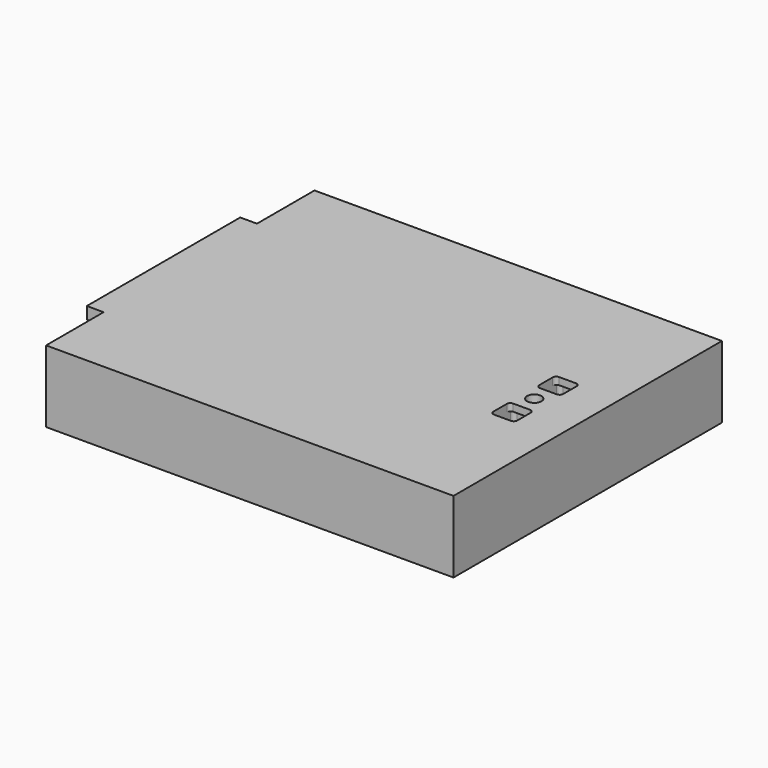
from build123d import *

# Parameters (mm, degrees)
F0_W     = 5
F0_H     = 24
F0_H_2   = 12
F0_R     = 2.55
F0_W_2   = 3
F1_DEPTH = 30
F2_START = -13
F2_DEPTH = 17
F3_START = -3
F3_DEPTH = 27
F4_START = -8
F4_DEPTH = 22
F5_DEPTH = 3
F6_DEPTH = 5


# Not quite as in the source:
# - a feature names something its author has since deleted; it is built from what else it names


with BuildPart() as f1:
    # F0 (on Top) → F1 (new body)
    with BuildSketch(Plane.XY):
        Polygon((82.5, 70), (-87.5, 70), (-87.5, 65), (-87.5, 40), (-87.5, 5), (-87.5, -5), (-87.5, -40), (-87.5, -65), (-87.5, -70), (-82.5, -70), (82.5, -70), (82.5, 0), align=None)
        Polygon((47.5, -65), (-82.5, -65), (-82.5, 65), (47.5, 65), (52.5, 65), (77.5, 65), (77.5, 0), (77.5, -65), (52.5, -65), align=None, mode=Mode.SUBTRACT)
        with BuildLine():
            Line((77.5, 65), (52.5, 65))
            Line((52.5, 65), (52.5, 41))
            Line((52.5, 41), (55.5, 41))
            Line((55.5, 41), (55.5, 44.499418828))
            ThreePointArc((55.5, 44.499418828), (55.9393398282, 45.5600789998), (57, 45.999418828))
            Line((57, 45.999418828), (63.8683293534, 45.999418828))
            ThreePointArc((63.8683293534, 45.999418828), (64.9248818439, 45.5641708343), (65.3682845321, 44.5110146078))
            Line((65.3682845321, 44.5110146078), (65.5, 27.4731523439))
            Line((65.5, 27.4731523439), (65.5, 18.9731523439))
            Line((65.5, 18.9731523439), (65.5, 17.4731523439))
            Line((65.5, 17.4731523439), (65.5, 16.9731523439))
            Line((65.5, 16.9731523439), (65.5, 15.4731523439))
            Line((65.5, 15.4731523439), (65.5, 8.4731523439))
            Line((65.5, 8.4731523439), (65.5, 6.9731523439))
            Line((65.5, 6.9731523439), (65.5, 6.4731523439))
            ThreePointArc((65.5, 6.4731523439), (65.0606601718, 5.4124921721), (64, 4.9731523439))
            Line((64, 4.9731523439), (57, 4.9731523439))
            ThreePointArc((57, 4.9731523439), (55.9393398282, 5.4124921721), (55.5, 6.4731523439))
            Line((55.5, 6.4731523439), (55.5, 6.9731523439))
            Line((55.5, 6.9731523439), (55.5, 8.4731523439))
            Line((55.5, 8.4731523439), (55.5, 15.4731523439))
            Line((55.5, 15.4731523439), (55.5, 16.9731523439))
            Line((55.5, 16.9731523439), (55.5, 17.4731523439))
            Line((55.5, 17.4731523439), (55.5, 18.9731523439))
            Line((55.5, 18.9731523439), (55.5, 27.4731523439))
            Line((55.5, 27.4731523439), (55.5, 29))
            Line((55.5, 29), (52.5, 29))
            Line((52.5, 29), (52.5, 0))
            Line((52.5, 0), (57.1866021752, 0))
            ThreePointArc((57.1866021752, 0), (60.1866021752, 3), (63.1866021752, 0))
            Line((63.1866021752, 0), (77.5, 0))
            Line((77.5, 0), (77.5, 65))
        make_face()
        with BuildLine():
            Line((52.5, -64.151630939), (52.5, -65))
            Line((52.5, -65), (77.5, -65))
            Line((77.5, -65), (77.5, 0))
            Line((77.5, 0), (63.1866021752, 0))
            ThreePointArc((63.1866021752, 0), (60.1866021752, -3), (57.1866021752, 0))
            Line((57.1866021752, 0), (52.5, 0))
            Line((52.5, 0), (52.5, -50))
            Line((52.5, -50), (55.5, -50))
            Line((55.5, -50), (55.5, -45))
            Line((55.5, -45), (55.5, -28.9731503129))
            Line((55.5, -28.9731503129), (55.5, -27.4731523439))
            Line((55.5, -27.4731523439), (55.5, -17.4731523439))
            Line((55.5, -17.4731523439), (55.5, -15.4731523439))
            Line((55.5, -15.4731523439), (55.5, -8.4731523439))
            Line((55.5, -8.4731523439), (55.5, -6.4731523439))
            ThreePointArc((55.5, -6.4731523439), (55.9393398282, -5.4124921721), (57, -4.9731523439))
            Line((57, -4.9731523439), (64, -4.9731523439))
            ThreePointArc((64, -4.9731523439), (65.0606601718, -5.4124921721), (65.5, -6.4731523439))
            Line((65.5, -6.4731523439), (65.5, -8.4731523439))
            Line((65.5, -8.4731523439), (65.5, -15.4731523439))
            Line((65.5, -15.4731523439), (65.5, -17.4731523439))
            Line((65.5, -17.4731523439), (65.5, -27.4731523439))
            Line((65.5, -27.4731523439), (65.4868731143, -29.171161501))
            Line((65.4868731143, -29.171161501), (65.3645118363, -44.9990261692))
            Line((65.3645118363, -44.9990261692), (65.3645118363, -51.4731504917))
            Line((65.3645118363, -51.4731504917), (65.3645118363, -58.4731504917))
            Line((65.3645118363, -58.4731504917), (65.3645118363, -62.651630939))
            ThreePointArc((65.3645118363, -62.651630939), (64.9251720081, -63.7122911108), (63.8645118363, -64.151630939))
            Line((63.8645118363, -64.151630939), (55.5, -64.151630939))
            Line((55.5, -64.151630939), (52.5, -64.151630939))
        make_face()
        Polygon((47.5, -0.9090909091), (47.5, -50), (52.5, -50), (52.5, 0), (52.5, 29), (47.5, 29), (47.5, 0.9090909091), align=None)
        with BuildLine():
            Line((55.5, 44.499418828), (55.5, 41))
            Line((55.5, 41), (55.5, 29))
            Line((55.5, 29), (55.5, 27.4731523439))
            Line((55.5, 27.4731523439), (55.5, 18.9731523439))
            Line((55.5, 18.9731523439), (57, 18.9731523439))
            Line((57, 18.9731523439), (64, 18.9731523439))
            Line((64, 18.9731523439), (65.5, 18.9731523439))
            Line((65.5, 18.9731523439), (65.5, 27.4731523439))
            Line((65.5, 27.4731523439), (65.3682845321, 44.5110146078))
            ThreePointArc((65.3682845321, 44.5110146078), (64.9248818439, 45.5641708343), (63.8683293534, 45.999418828))
            Line((63.8683293534, 45.999418828), (57, 45.999418828))
            ThreePointArc((57, 45.999418828), (55.9393398282, 45.5600789998), (55.5, 44.499418828))
        make_face()
        Polygon((60.6, 20.97), (56.5, 23.8318176043), (56.5, 28.1081823957), (60.6, 30.97), (64.7, 28.1081823957), (64.7, 23.8318176043), align=None, mode=Mode.SUBTRACT)
        with BuildLine():
            Line((55.5, -45), (55.5, -50))
            Line((55.5, -50), (57, -49.9731504917))
            Line((57, -49.9731504917), (63.8645118363, -49.9731504917))
            ThreePointArc((63.8645118363, -49.9731504917), (64.9251720081, -50.4124903199), (65.3645118363, -51.4731504917))
            Line((65.3645118363, -51.4731504917), (65.3645118363, -44.9990261692))
            Line((65.3645118363, -44.9990261692), (65.4868731143, -29.171161501))
            ThreePointArc((65.4868731143, -29.171161501), (64.9881759296, -30.1016486032), (64.0000000298, -30.4731503129))
            Line((64.0000000298, -30.4731503129), (57.0000000298, -30.4731503129))
            ThreePointArc((57.0000000298, -30.4731503129), (55.939339858, -30.0338104847), (55.5000000298, -28.9731503129))
            Line((55.5, -28.9731503129), (55.5, -45))
        make_face()
        with BuildLine():
            Line((55.5, -58.4731504917), (55.5, -64.151630939))
            Line((55.5, -64.151630939), (63.8645118363, -64.151630939))
            ThreePointArc((63.8645118363, -64.151630939), (64.9251720081, -63.7122911108), (65.3645118363, -62.651630939))
            Line((65.3645118363, -62.651630939), (65.3645118363, -58.4731504917))
            Line((65.3645118363, -58.4731504917), (65.3645118363, -51.4731504917))
            ThreePointArc((65.3645118363, -51.4731504917), (64.9251720081, -50.4124903199), (63.8645118363, -49.9731504917))
            Line((63.8645118363, -49.9731504917), (57, -49.9731504917))
            Line((57, -49.9731504917), (55.5, -50))
            Line((55.5, -50), (55.5, -51.4731504917))
            Line((55.5, -51.4731504917), (55.5, -58.4731504917))
        make_face()
        Polygon((60.4814975321, -60.5032157659), (56.3814975321, -57.6413981616), (56.3814975321, -53.3650333702), (60.4814975321, -50.5032157659), (64.5814975321, -53.3650333702), (64.5814975321, -57.6413981616), align=None, mode=Mode.SUBTRACT)
        with Locations((50, 53)):
            Rectangle(F0_W, F0_H)
        with BuildLine():
            Line((55.5, -27.4731523439), (55.5, -28.9731503129))
            ThreePointArc((55.5000000298, -28.9731503129), (55.939339858, -30.0338104847), (57.0000000298, -30.4731503129))
            Line((57.0000000298, -30.4731503129), (64.0000000298, -30.4731503129))
            ThreePointArc((64.0000000298, -30.4731503129), (64.9881759296, -30.1016486032), (65.4868731143, -29.171161501))
            Line((65.4868731143, -29.171161501), (65.5, -27.4731523439))
            Line((65.5, -27.4731523439), (65.5, -17.4731523439))
            ThreePointArc((65.5, -17.4731523439), (65.0606601718, -18.5338125156), (64, -18.9731523439))
            Line((64, -18.9731523439), (57, -18.9731523439))
            ThreePointArc((57, -18.9731523439), (55.9393398282, -18.5338125156), (55.5, -17.4731523439))
            Line((55.5, -17.4731523439), (55.5, -27.4731523439))
        make_face()
        Polygon((60.6000007153, -29.9631433734), (56.5000007153, -27.1013257692), (56.5000007153, -22.8249609777), (60.6000007153, -19.9631433734), (64.7000007153, -22.8249609777), (64.7000007153, -27.1013257692), align=None, mode=Mode.SUBTRACT)
        Polygon((47.5, -50), (47.5, -65), (52.5, -65), (52.5, -64.151630939), (52.5, -50), align=None)
        with Locations((50, 35)):
            Rectangle(F0_W, F0_H_2)
        Polygon((56.5, 28.1081823957), (56.5, 23.8318176043), (60.6, 20.97), (64.7, 23.8318176043), (64.7, 28.1081823957), (60.6, 30.97), align=None)
        with Locations((60.6, 25.9731523439)):
            Circle(F0_R, mode=Mode.SUBTRACT)
        Polygon((56.3814975321, -53.3650333702), (56.3814975321, -57.6413981616), (60.4814975321, -60.5032157659), (64.5814975321, -57.6413981616), (64.5814975321, -53.3650333702), (60.4814975321, -50.5032157659), align=None)
        with Locations((60.4823811061, -55.5000021935)):
            Circle(F0_R, mode=Mode.SUBTRACT)
        Polygon((56.5000007153, -22.8249609777), (56.5000007153, -27.1013257692), (60.6000007153, -29.9631433734), (64.7000007153, -27.1013257692), (64.7000007153, -22.8249609777), (60.6000007153, -19.9631433734), align=None)
        with Locations((60.6000007153, -24.9631504917)):
            Circle(F0_R, mode=Mode.SUBTRACT)
        Polygon((52.5, -50), (52.5, -64.151630939), (55.5, -64.151630939), (55.5, -58.4731504917), (55.5, -51.4731504917), (55.5, -50), align=None)
        with Locations((54, 35)):
            Rectangle(F0_W_2, F0_H_2)
        with Locations((60.6000007153, -24.9631504917)):
            Circle(F0_R)
        with Locations((60.4823811061, -55.5000021935)):
            Circle(F0_R)
        with Locations((60.6, 25.9731523439)):
            Circle(F0_R)
        with BuildLine():
            Line((55.5, -6.4731523439), (55.5, -8.4731523439))
            ThreePointArc((55.5, -8.4731523439), (55.9393398282, -7.4124921721), (57, -6.9731523439))
            Line((57, -6.9731523439), (64, -6.9731523439))
            ThreePointArc((64, -6.9731523439), (65.0606601718, -7.4124921721), (65.5, -8.4731523439))
            Line((65.5, -8.4731523439), (65.5, -6.4731523439))
            ThreePointArc((65.5, -6.4731523439), (65.0606601718, -5.4124921721), (64, -4.9731523439))
            Line((64, -4.9731523439), (57, -4.9731523439))
            ThreePointArc((57, -4.9731523439), (55.9393398282, -5.4124921721), (55.5, -6.4731523439))
        make_face()
        with BuildLine():
            Line((55.5, -15.4731523439), (55.5, -17.4731523439))
            ThreePointArc((55.5, -17.4731523439), (55.9393398282, -18.5338125156), (57, -18.9731523439))
            Line((57, -18.9731523439), (64, -18.9731523439))
            ThreePointArc((64, -18.9731523439), (65.0606601718, -18.5338125156), (65.5, -17.4731523439))
            Line((65.5, -17.4731523439), (65.5, -15.4731523439))
            ThreePointArc((65.5, -15.4731523439), (65.0606601718, -16.5338125156), (64, -16.9731523439))
            Line((64, -16.9731523439), (57, -16.9731523439))
            ThreePointArc((57, -16.9731523439), (55.9393398282, -16.5338125156), (55.5, -15.4731523439))
        make_face()
        with BuildLine():
            Line((64, 18.9731523439), (57, 18.9731523439))
            ThreePointArc((57, 18.9731523439), (55.9393398282, 18.5338125156), (55.5, 17.4731523439))
            Line((55.5, 17.4731523439), (55.5, 16.9731523439))
            Line((55.5, 16.9731523439), (57, 16.9731523439))
            Line((57, 16.9731523439), (64, 16.9731523439))
            Line((64, 16.9731523439), (65.5, 16.9731523439))
            Line((65.5, 16.9731523439), (65.5, 17.4731523439))
            ThreePointArc((65.5, 17.4731523439), (65.0606601718, 18.5338125156), (64, 18.9731523439))
        make_face()
        with BuildLine():
            Line((57, 6.9731523439), (55.5, 6.9731523439))
            Line((55.5, 6.9731523439), (55.5, 6.4731523439))
            ThreePointArc((55.5, 6.4731523439), (55.9393398282, 5.4124921721), (57, 4.9731523439))
            Line((57, 4.9731523439), (64, 4.9731523439))
            ThreePointArc((64, 4.9731523439), (65.0606601718, 5.4124921721), (65.5, 6.4731523439))
            Line((65.5, 6.4731523439), (65.5, 6.9731523439))
            Line((65.5, 6.9731523439), (64, 6.9731523439))
            Line((64, 6.9731523439), (57, 6.9731523439))
        make_face()
        with BuildLine():
            Line((65.5, 18.9731523439), (64, 18.9731523439))
            ThreePointArc((64, 18.9731523439), (65.0606601718, 18.5338125156), (65.5, 17.4731523439))
            Line((65.5, 17.4731523439), (65.5, 18.9731523439))
        make_face()
        with BuildLine():
            Line((57, 18.9731523439), (55.5, 18.9731523439))
            Line((55.5, 18.9731523439), (55.5, 17.4731523439))
            ThreePointArc((55.5, 17.4731523439), (55.9393398282, 18.5338125156), (57, 18.9731523439))
        make_face()
        with BuildLine():
            Line((57, 16.9731523439), (55.5, 16.9731523439))
            Line((55.5, 16.9731523439), (55.5, 15.4731523439))
            ThreePointArc((55.5, 15.4731523439), (55.9393398282, 16.5338125156), (57, 16.9731523439))
        make_face()
        with BuildLine():
            Line((65.5, 15.4731523439), (65.5, 16.9731523439))
            Line((65.5, 16.9731523439), (64, 16.9731523439))
            ThreePointArc((64, 16.9731523439), (65.0606601718, 16.5338125156), (65.5, 15.4731523439))
        make_face()
        with BuildLine():
            Line((65.5, 6.9731523439), (65.5, 8.4731523439))
            ThreePointArc((65.5, 8.4731523439), (65.0606601718, 7.4124921721), (64, 6.9731523439))
            Line((64, 6.9731523439), (65.5, 6.9731523439))
        make_face()
        with BuildLine():
            ThreePointArc((57, 6.9731523439), (55.9393398282, 7.4124921721), (55.5, 8.4731523439))
            Line((55.5, 8.4731523439), (55.5, 6.9731523439))
            Line((55.5, 6.9731523439), (57, 6.9731523439))
        make_face()
    extrude(amount=-F1_DEPTH)

    # F0 (on Top) → F2 (cut)
    with BuildSketch(Plane.XY.offset(F2_START)):
        with BuildLine():
            Line((77.5, 65), (52.5, 65))
            Line((52.5, 65), (52.5, 41))
            Line((52.5, 41), (55.5, 41))
            Line((55.5, 41), (55.5, 44.499418828))
            ThreePointArc((55.5, 44.499418828), (55.9393398282, 45.5600789998), (57, 45.999418828))
            Line((57, 45.999418828), (63.8683293534, 45.999418828))
            ThreePointArc((63.8683293534, 45.999418828), (64.9248818439, 45.5641708343), (65.3682845321, 44.5110146078))
            Line((65.3682845321, 44.5110146078), (65.5, 27.4731523439))
            Line((65.5, 27.4731523439), (65.5, 18.9731523439))
            Line((65.5, 18.9731523439), (65.5, 17.4731523439))
            Line((65.5, 17.4731523439), (65.5, 16.9731523439))
            Line((65.5, 16.9731523439), (65.5, 15.4731523439))
            Line((65.5, 15.4731523439), (65.5, 8.4731523439))
            Line((65.5, 8.4731523439), (65.5, 6.9731523439))
            Line((65.5, 6.9731523439), (65.5, 6.4731523439))
            ThreePointArc((65.5, 6.4731523439), (65.0606601718, 5.4124921721), (64, 4.9731523439))
            Line((64, 4.9731523439), (57, 4.9731523439))
            ThreePointArc((57, 4.9731523439), (55.9393398282, 5.4124921721), (55.5, 6.4731523439))
            Line((55.5, 6.4731523439), (55.5, 6.9731523439))
            Line((55.5, 6.9731523439), (55.5, 8.4731523439))
            Line((55.5, 8.4731523439), (55.5, 15.4731523439))
            Line((55.5, 15.4731523439), (55.5, 16.9731523439))
            Line((55.5, 16.9731523439), (55.5, 17.4731523439))
            Line((55.5, 17.4731523439), (55.5, 18.9731523439))
            Line((55.5, 18.9731523439), (55.5, 27.4731523439))
            Line((55.5, 27.4731523439), (55.5, 29))
            Line((55.5, 29), (52.5, 29))
            Line((52.5, 29), (52.5, 0))
            Line((52.5, 0), (57.1866021752, 0))
            ThreePointArc((57.1866021752, 0), (60.1866021752, 3), (63.1866021752, 0))
            Line((63.1866021752, 0), (77.5, 0))
            Line((77.5, 0), (77.5, 65))
        make_face()
        with BuildLine():
            Line((52.5, -64.151630939), (52.5, -65))
            Line((52.5, -65), (77.5, -65))
            Line((77.5, -65), (77.5, 0))
            Line((77.5, 0), (63.1866021752, 0))
            ThreePointArc((63.1866021752, 0), (60.1866021752, -3), (57.1866021752, 0))
            Line((57.1866021752, 0), (52.5, 0))
            Line((52.5, 0), (52.5, -50))
            Line((52.5, -50), (55.5, -50))
            Line((55.5, -50), (55.5, -45))
            Line((55.5, -45), (55.5, -28.9731503129))
            Line((55.5, -28.9731503129), (55.5, -27.4731523439))
            Line((55.5, -27.4731523439), (55.5, -17.4731523439))
            Line((55.5, -17.4731523439), (55.5, -15.4731523439))
            Line((55.5, -15.4731523439), (55.5, -8.4731523439))
            Line((55.5, -8.4731523439), (55.5, -6.4731523439))
            ThreePointArc((55.5, -6.4731523439), (55.9393398282, -5.4124921721), (57, -4.9731523439))
            Line((57, -4.9731523439), (64, -4.9731523439))
            ThreePointArc((64, -4.9731523439), (65.0606601718, -5.4124921721), (65.5, -6.4731523439))
            Line((65.5, -6.4731523439), (65.5, -8.4731523439))
            Line((65.5, -8.4731523439), (65.5, -15.4731523439))
            Line((65.5, -15.4731523439), (65.5, -17.4731523439))
            Line((65.5, -17.4731523439), (65.5, -27.4731523439))
            Line((65.5, -27.4731523439), (65.4868731143, -29.171161501))
            Line((65.4868731143, -29.171161501), (65.3645118363, -44.9990261692))
            Line((65.3645118363, -44.9990261692), (65.3645118363, -51.4731504917))
            Line((65.3645118363, -51.4731504917), (65.3645118363, -58.4731504917))
            Line((65.3645118363, -58.4731504917), (65.3645118363, -62.651630939))
            ThreePointArc((65.3645118363, -62.651630939), (64.9251720081, -63.7122911108), (63.8645118363, -64.151630939))
            Line((63.8645118363, -64.151630939), (55.5, -64.151630939))
            Line((55.5, -64.151630939), (52.5, -64.151630939))
        make_face()
        with Locations((50, 53)):
            Rectangle(F0_W, F0_H)
    extrude(amount=-F2_DEPTH, mode=Mode.SUBTRACT)

    # F0 (on Top) → F3 (cut)
    with BuildSketch(Plane.XY.offset(F3_START)):
        with BuildLine():
            Line((64, 18.9731523439), (57, 18.9731523439))
            ThreePointArc((57, 18.9731523439), (55.9393398282, 18.5338125156), (55.5, 17.4731523439))
            Line((55.5, 17.4731523439), (55.5, 16.9731523439))
            Line((55.5, 16.9731523439), (57, 16.9731523439))
            Line((57, 16.9731523439), (64, 16.9731523439))
            Line((64, 16.9731523439), (65.5, 16.9731523439))
            Line((65.5, 16.9731523439), (65.5, 17.4731523439))
            ThreePointArc((65.5, 17.4731523439), (65.0606601718, 18.5338125156), (64, 18.9731523439))
        make_face()
        with BuildLine():
            Line((57, 6.9731523439), (55.5, 6.9731523439))
            Line((55.5, 6.9731523439), (55.5, 6.4731523439))
            ThreePointArc((55.5, 6.4731523439), (55.9393398282, 5.4124921721), (57, 4.9731523439))
            Line((57, 4.9731523439), (64, 4.9731523439))
            ThreePointArc((64, 4.9731523439), (65.0606601718, 5.4124921721), (65.5, 6.4731523439))
            Line((65.5, 6.4731523439), (65.5, 6.9731523439))
            Line((65.5, 6.9731523439), (64, 6.9731523439))
            Line((64, 6.9731523439), (57, 6.9731523439))
        make_face()
        with BuildLine():
            Line((57, 16.9731523439), (55.5, 16.9731523439))
            Line((55.5, 16.9731523439), (55.5, 15.4731523439))
            ThreePointArc((55.5, 15.4731523439), (55.9393398282, 16.5338125156), (57, 16.9731523439))
        make_face()
        with BuildLine():
            Line((65.5, 15.4731523439), (65.5, 16.9731523439))
            Line((65.5, 16.9731523439), (64, 16.9731523439))
            ThreePointArc((64, 16.9731523439), (65.0606601718, 16.5338125156), (65.5, 15.4731523439))
        make_face()
        with BuildLine():
            Line((65.5, 6.9731523439), (65.5, 8.4731523439))
            ThreePointArc((65.5, 8.4731523439), (65.0606601718, 7.4124921721), (64, 6.9731523439))
            Line((64, 6.9731523439), (65.5, 6.9731523439))
        make_face()
        with BuildLine():
            ThreePointArc((57, 6.9731523439), (55.9393398282, 7.4124921721), (55.5, 8.4731523439))
            Line((55.5, 8.4731523439), (55.5, 6.9731523439))
            Line((55.5, 6.9731523439), (57, 6.9731523439))
        make_face()
        with BuildLine():
            Line((55.5, -6.4731523439), (55.5, -8.4731523439))
            ThreePointArc((55.5, -8.4731523439), (55.9393398282, -7.4124921721), (57, -6.9731523439))
            Line((57, -6.9731523439), (64, -6.9731523439))
            ThreePointArc((64, -6.9731523439), (65.0606601718, -7.4124921721), (65.5, -8.4731523439))
            Line((65.5, -8.4731523439), (65.5, -6.4731523439))
            ThreePointArc((65.5, -6.4731523439), (65.0606601718, -5.4124921721), (64, -4.9731523439))
            Line((64, -4.9731523439), (57, -4.9731523439))
            ThreePointArc((57, -4.9731523439), (55.9393398282, -5.4124921721), (55.5, -6.4731523439))
        make_face()
        with BuildLine():
            Line((55.5, -15.4731523439), (55.5, -17.4731523439))
            ThreePointArc((55.5, -17.4731523439), (55.9393398282, -18.5338125156), (57, -18.9731523439))
            Line((57, -18.9731523439), (64, -18.9731523439))
            ThreePointArc((64, -18.9731523439), (65.0606601718, -18.5338125156), (65.5, -17.4731523439))
            Line((65.5, -17.4731523439), (65.5, -15.4731523439))
            ThreePointArc((65.5, -15.4731523439), (65.0606601718, -16.5338125156), (64, -16.9731523439))
            Line((64, -16.9731523439), (57, -16.9731523439))
            ThreePointArc((57, -16.9731523439), (55.9393398282, -16.5338125156), (55.5, -15.4731523439))
        make_face()
        Polygon((56.3814975321, -53.3650333702), (56.3814975321, -57.6413981616), (60.4814975321, -60.5032157659), (64.5814975321, -57.6413981616), (64.5814975321, -53.3650333702), (60.4814975321, -50.5032157659), align=None)
        with Locations((60.4823811061, -55.5000021935)):
            Circle(F0_R, mode=Mode.SUBTRACT)
        Polygon((56.5000007153, -22.8249609777), (56.5000007153, -27.1013257692), (60.6000007153, -29.9631433734), (64.7000007153, -27.1013257692), (64.7000007153, -22.8249609777), (60.6000007153, -19.9631433734), align=None)
        with Locations((60.6000007153, -24.9631504917)):
            Circle(F0_R, mode=Mode.SUBTRACT)
        with Locations((60.6000007153, -24.9631504917)):
            Circle(F0_R)
        with Locations((60.4823811061, -55.5000021935)):
            Circle(F0_R)
        with BuildLine():
            Line((55.5, -45), (55.5, -50))
            Line((55.5, -50), (57, -49.9731504917))
            Line((57, -49.9731504917), (63.8645118363, -49.9731504917))
            ThreePointArc((63.8645118363, -49.9731504917), (64.9251720081, -50.4124903199), (65.3645118363, -51.4731504917))
            Line((65.3645118363, -51.4731504917), (65.3645118363, -44.9990261692))
            Line((65.3645118363, -44.9990261692), (65.4868731143, -29.171161501))
            ThreePointArc((65.4868731143, -29.171161501), (64.9881759296, -30.1016486032), (64.0000000298, -30.4731503129))
            Line((64.0000000298, -30.4731503129), (57.0000000298, -30.4731503129))
            ThreePointArc((57.0000000298, -30.4731503129), (55.939339858, -30.0338104847), (55.5000000298, -28.9731503129))
            Line((55.5, -28.9731503129), (55.5, -45))
        make_face()
        Polygon((56.5, 28.1081823957), (56.5, 23.8318176043), (60.6, 20.97), (64.7, 23.8318176043), (64.7, 28.1081823957), (60.6, 30.97), align=None)
        with Locations((60.6, 25.9731523439)):
            Circle(F0_R, mode=Mode.SUBTRACT)
        with Locations((60.6, 25.9731523439)):
            Circle(F0_R)
    extrude(amount=-F3_DEPTH, mode=Mode.SUBTRACT)

    # F0 (on Top) → F4 (cut)
    with BuildSketch(Plane.XY.offset(F4_START)):
        with BuildLine():
            Line((55.5, 44.499418828), (55.5, 41))
            Line((55.5, 41), (55.5, 29))
            Line((55.5, 29), (55.5, 27.4731523439))
            Line((55.5, 27.4731523439), (55.5, 18.9731523439))
            Line((55.5, 18.9731523439), (57, 18.9731523439))
            Line((57, 18.9731523439), (64, 18.9731523439))
            Line((64, 18.9731523439), (65.5, 18.9731523439))
            Line((65.5, 18.9731523439), (65.5, 27.4731523439))
            Line((65.5, 27.4731523439), (65.3682845321, 44.5110146078))
            ThreePointArc((65.3682845321, 44.5110146078), (64.9248818439, 45.5641708343), (63.8683293534, 45.999418828))
            Line((63.8683293534, 45.999418828), (57, 45.999418828))
            ThreePointArc((57, 45.999418828), (55.9393398282, 45.5600789998), (55.5, 44.499418828))
        make_face()
        Polygon((60.6, 20.97), (56.5, 23.8318176043), (56.5, 28.1081823957), (60.6, 30.97), (64.7, 28.1081823957), (64.7, 23.8318176043), align=None, mode=Mode.SUBTRACT)
        with BuildLine():
            Line((65.5, 18.9731523439), (64, 18.9731523439))
            ThreePointArc((64, 18.9731523439), (65.0606601718, 18.5338125156), (65.5, 17.4731523439))
            Line((65.5, 17.4731523439), (65.5, 18.9731523439))
        make_face()
        with BuildLine():
            Line((57, 18.9731523439), (55.5, 18.9731523439))
            Line((55.5, 18.9731523439), (55.5, 17.4731523439))
            ThreePointArc((55.5, 17.4731523439), (55.9393398282, 18.5338125156), (57, 18.9731523439))
        make_face()
        with BuildLine():
            Line((64, 18.9731523439), (57, 18.9731523439))
            ThreePointArc((57, 18.9731523439), (55.9393398282, 18.5338125156), (55.5, 17.4731523439))
            Line((55.5, 17.4731523439), (55.5, 16.9731523439))
            Line((55.5, 16.9731523439), (57, 16.9731523439))
            Line((57, 16.9731523439), (64, 16.9731523439))
            Line((64, 16.9731523439), (65.5, 16.9731523439))
            Line((65.5, 16.9731523439), (65.5, 17.4731523439))
            ThreePointArc((65.5, 17.4731523439), (65.0606601718, 18.5338125156), (64, 18.9731523439))
        make_face()
        with BuildLine():
            Line((57, 6.9731523439), (55.5, 6.9731523439))
            Line((55.5, 6.9731523439), (55.5, 6.4731523439))
            ThreePointArc((55.5, 6.4731523439), (55.9393398282, 5.4124921721), (57, 4.9731523439))
            Line((57, 4.9731523439), (64, 4.9731523439))
            ThreePointArc((64, 4.9731523439), (65.0606601718, 5.4124921721), (65.5, 6.4731523439))
            Line((65.5, 6.4731523439), (65.5, 6.9731523439))
            Line((65.5, 6.9731523439), (64, 6.9731523439))
            Line((64, 6.9731523439), (57, 6.9731523439))
        make_face()
        with BuildLine():
            Line((55.5, -6.4731523439), (55.5, -8.4731523439))
            ThreePointArc((55.5, -8.4731523439), (55.9393398282, -7.4124921721), (57, -6.9731523439))
            Line((57, -6.9731523439), (64, -6.9731523439))
            ThreePointArc((64, -6.9731523439), (65.0606601718, -7.4124921721), (65.5, -8.4731523439))
            Line((65.5, -8.4731523439), (65.5, -6.4731523439))
            ThreePointArc((65.5, -6.4731523439), (65.0606601718, -5.4124921721), (64, -4.9731523439))
            Line((64, -4.9731523439), (57, -4.9731523439))
            ThreePointArc((57, -4.9731523439), (55.9393398282, -5.4124921721), (55.5, -6.4731523439))
        make_face()
        with BuildLine():
            Line((55.5, -15.4731523439), (55.5, -17.4731523439))
            ThreePointArc((55.5, -17.4731523439), (55.9393398282, -18.5338125156), (57, -18.9731523439))
            Line((57, -18.9731523439), (64, -18.9731523439))
            ThreePointArc((64, -18.9731523439), (65.0606601718, -18.5338125156), (65.5, -17.4731523439))
            Line((65.5, -17.4731523439), (65.5, -15.4731523439))
            ThreePointArc((65.5, -15.4731523439), (65.0606601718, -16.5338125156), (64, -16.9731523439))
            Line((64, -16.9731523439), (57, -16.9731523439))
            ThreePointArc((57, -16.9731523439), (55.9393398282, -16.5338125156), (55.5, -15.4731523439))
        make_face()
        with BuildLine():
            Line((55.5, -27.4731523439), (55.5, -28.9731503129))
            ThreePointArc((55.5000000298, -28.9731503129), (55.939339858, -30.0338104847), (57.0000000298, -30.4731503129))
            Line((57.0000000298, -30.4731503129), (64.0000000298, -30.4731503129))
            ThreePointArc((64.0000000298, -30.4731503129), (64.9881759296, -30.1016486032), (65.4868731143, -29.171161501))
            Line((65.4868731143, -29.171161501), (65.5, -27.4731523439))
            Line((65.5, -27.4731523439), (65.5, -17.4731523439))
            ThreePointArc((65.5, -17.4731523439), (65.0606601718, -18.5338125156), (64, -18.9731523439))
            Line((64, -18.9731523439), (57, -18.9731523439))
            ThreePointArc((57, -18.9731523439), (55.9393398282, -18.5338125156), (55.5, -17.4731523439))
            Line((55.5, -17.4731523439), (55.5, -27.4731523439))
        make_face()
        Polygon((60.6000007153, -29.9631433734), (56.5000007153, -27.1013257692), (56.5000007153, -22.8249609777), (60.6000007153, -19.9631433734), (64.7000007153, -22.8249609777), (64.7000007153, -27.1013257692), align=None, mode=Mode.SUBTRACT)
        Polygon((52.5, -50), (52.5, -64.151630939), (55.5, -64.151630939), (55.5, -58.4731504917), (55.5, -51.4731504917), (55.5, -50), align=None)
        Polygon((47.5, -50), (47.5, -65), (52.5, -65), (52.5, -64.151630939), (52.5, -50), align=None)
        with Locations((54, 35)):
            Rectangle(F0_W_2, F0_H_2)
        with Locations((50, 35)):
            Rectangle(F0_W, F0_H_2)
        with BuildLine():
            Line((55.5, -58.4731504917), (55.5, -64.151630939))
            Line((55.5, -64.151630939), (63.8645118363, -64.151630939))
            ThreePointArc((63.8645118363, -64.151630939), (64.9251720081, -63.7122911108), (65.3645118363, -62.651630939))
            Line((65.3645118363, -62.651630939), (65.3645118363, -58.4731504917))
            Line((65.3645118363, -58.4731504917), (65.3645118363, -51.4731504917))
            ThreePointArc((65.3645118363, -51.4731504917), (64.9251720081, -50.4124903199), (63.8645118363, -49.9731504917))
            Line((63.8645118363, -49.9731504917), (57, -49.9731504917))
            Line((57, -49.9731504917), (55.5, -50))
            Line((55.5, -50), (55.5, -51.4731504917))
            Line((55.5, -51.4731504917), (55.5, -58.4731504917))
        make_face()
        Polygon((60.4814975321, -60.5032157659), (56.3814975321, -57.6413981616), (56.3814975321, -53.3650333702), (60.4814975321, -50.5032157659), (64.5814975321, -53.3650333702), (64.5814975321, -57.6413981616), align=None, mode=Mode.SUBTRACT)
    extrude(amount=-F4_DEPTH, mode=Mode.SUBTRACT)

    # F0 (on Top) → F5 (join)
    with BuildSketch(Plane.XY):
        Polygon((-82.5, 65), (-82.5, -65), (47.5, -65), (47.5, -50), (47.5, -0.9090909091), (47.5, 0.9090909091), (47.5, 29), (47.5, 41), (47.5, 65), align=None)
    extrude(amount=-F5_DEPTH)

    # F0 (on Top) → F6 (join)
    with BuildSketch(Plane.XY):
        Polygon((-87.5, 5), (-87.5, 40), (-94.5, 40), (-94.5, -40), (-87.5, -40), (-87.5, -5), align=None)
    extrude(amount=-F6_DEPTH)


solid = f1.part
